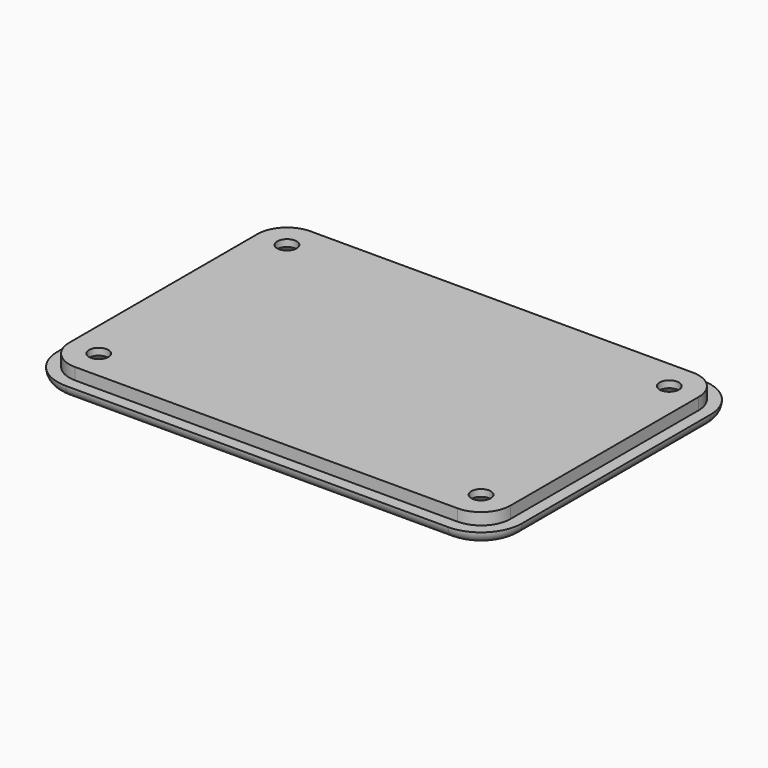
from build123d import *

# Parameters (mm, degrees)
F1_DEPTH       = 2
F2_DEPTH       = 4
F3_R           = 1.99999
F4_D           = 3.3
F4_CSINK_D     = 8.96
F4_CSINK_ANGLE = 90


# Not quite as in the source:
# - a fillet or chamfer is up to 0.001 mm smaller than in the source, because OpenCascade refuses the exact size


with BuildPart() as f1:
    # F0 (on Top) → F1 (new body)
    with BuildSketch(Plane.XY):
        with BuildLine():
            Line((32.5, 26.9999996311), (-32.5, 26.9999996311))
            ThreePointArc((-32.5, 26.9999996311), (-37.4497472074, 24.9497472074), (-39.4999996311, 20))
            Line((-39.4999996311, 20), (-39.4999996311, -20))
            ThreePointArc((-39.4999996311, -20), (-37.4497472074, -24.9497472074), (-32.5, -26.9999996311))
            Line((-32.5, -26.9999996311), (32.5, -26.9999996311))
            ThreePointArc((32.5, -26.9999996311), (37.4497472074, -24.9497472074), (39.4999996311, -20))
            Line((39.4999996311, -20), (39.4999996311, 20))
            ThreePointArc((39.4999996311, 20), (37.4497472074, 24.9497472074), (32.5, 26.9999996311))
        make_face()
        with BuildLine():
            ThreePointArc((-37.5, 20), (-36.0355339059, 23.5355339059), (-32.5, 25))
            Line((-32.5, 25), (32.5, 25))
            ThreePointArc((32.5, 25), (36.0355339059, 23.5355339059), (37.5, 20))
            Line((37.5, 20), (37.5, -20))
            ThreePointArc((37.5, -20), (36.0355339059, -23.5355339059), (32.5, -25))
            Line((32.5, -25), (-32.5, -25))
            ThreePointArc((-32.5, -25), (-36.0355339059, -23.5355339059), (-37.5, -20))
            Line((-37.5, -20), (-37.5, 20))
        make_face(mode=Mode.SUBTRACT)
        with BuildLine():
            Line((32.5, 25), (-32.5, 25))
            ThreePointArc((-32.5, 25), (-36.0355339059, 23.5355339059), (-37.5, 20))
            Line((-37.5, 20), (-37.5, -20))
            ThreePointArc((-37.5, -20), (-36.0355339059, -23.5355339059), (-32.5, -25))
            Line((-32.5, -25), (32.5, -25))
            ThreePointArc((32.5, -25), (36.0355339059, -23.5355339059), (37.5, -20))
            Line((37.5, -20), (37.5, 20))
            ThreePointArc((37.5, 20), (36.0355339059, 23.5355339059), (32.5, 25))
        make_face()
    extrude(amount=F1_DEPTH)

    # F0 (on Top) → F2 (join)
    with BuildSketch(Plane.XY):
        with BuildLine():
            Line((32.5, 25), (-32.5, 25))
            ThreePointArc((-32.5, 25), (-36.0355339059, 23.5355339059), (-37.5, 20))
            Line((-37.5, 20), (-37.5, -20))
            ThreePointArc((-37.5, -20), (-36.0355339059, -23.5355339059), (-32.5, -25))
            Line((-32.5, -25), (32.5, -25))
            ThreePointArc((32.5, -25), (36.0355339059, -23.5355339059), (37.5, -20))
            Line((37.5, -20), (37.5, 20))
            ThreePointArc((37.5, 20), (36.0355339059, 23.5355339059), (32.5, 25))
        make_face()
    extrude(amount=F2_DEPTH)

    # F3 (radius 2 in the source; OpenCascade refuses exactly that, so slightly less here)
    f3_edges = [f1.edges().sort_by_distance(p)[0] for p in [
        (0, 27, 0),
        (-37.449747, 24.949747, 0),
        (-39.5, 0, 0),
        (-37.449747, -24.949747, 0),
        (0, -27, 0),
        (37.449747, -24.949747, 0),
        (39.5, 0, 0),
        (37.449747, 24.949747, 0),
    ]]
    fillet(f3_edges, radius=F3_R)

    # F4 (through all)
    with Locations(Plane(origin=(0, 0, 0), x_dir=(1, 0, 0), z_dir=(0, 0, -1))):
        with Locations((32.5, 20), (32.5, -20), (-32.5, -20), (-32.5, 20)):
            CounterSinkHole(F4_D / 2, F4_CSINK_D / 2, counter_sink_angle=F4_CSINK_ANGLE)


solid = f1.part
